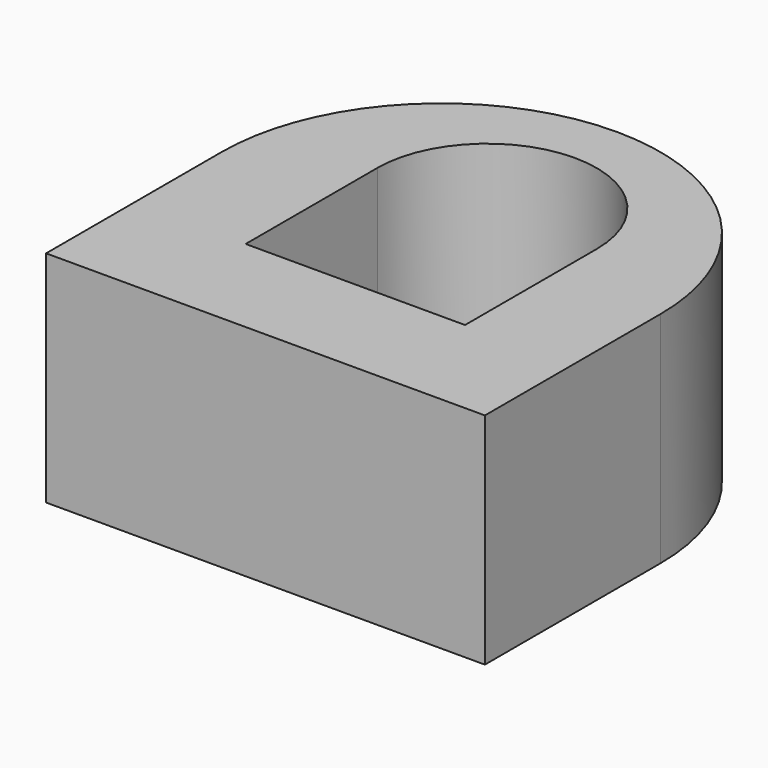
from build123d import *

# Parameters (mm, degrees)
F0_W     = 8
F0_H     = 8
F1_DEPTH = 4
F2_R     = 4
F3_R     = 3.99999


# Not quite as in the source:
# - a fillet or chamfer is up to 0.001 mm smaller than in the source, because OpenCascade refuses the exact size


with BuildPart() as f1:
    # F0 (on Top) → F1 (new body)
    with BuildSketch(Plane.XY):
        Rectangle(F0_W, F0_H)
        with BuildLine():
            Line((-1.9619476116, -2), (-1.9619476116, 1))
            ThreePointArc((-1.9619476116, 1), (0.0380527829, 2.9999996055), (2.0380523884, 0.9999992109))
            Line((2.0380523884, 0.9999992109), (2.0380523884, -2))
            Line((2.0380523884, -2), (-1.9619476116, -2))
        make_face(mode=Mode.SUBTRACT)
    extrude(amount=F1_DEPTH)

    # F2
    f2_edges = [f1.edges().sort_by_distance(p)[0] for p in [
        (4, 4, 2),
    ]]
    fillet(f2_edges, radius=F2_R)

    # F3 (radius 4 in the source; OpenCascade refuses exactly that, so slightly less here)
    f3_edges = [f1.edges().sort_by_distance(p)[0] for p in [
        (-4, 4, 2),
    ]]
    fillet(f3_edges, radius=F3_R)


solid = f1.part
